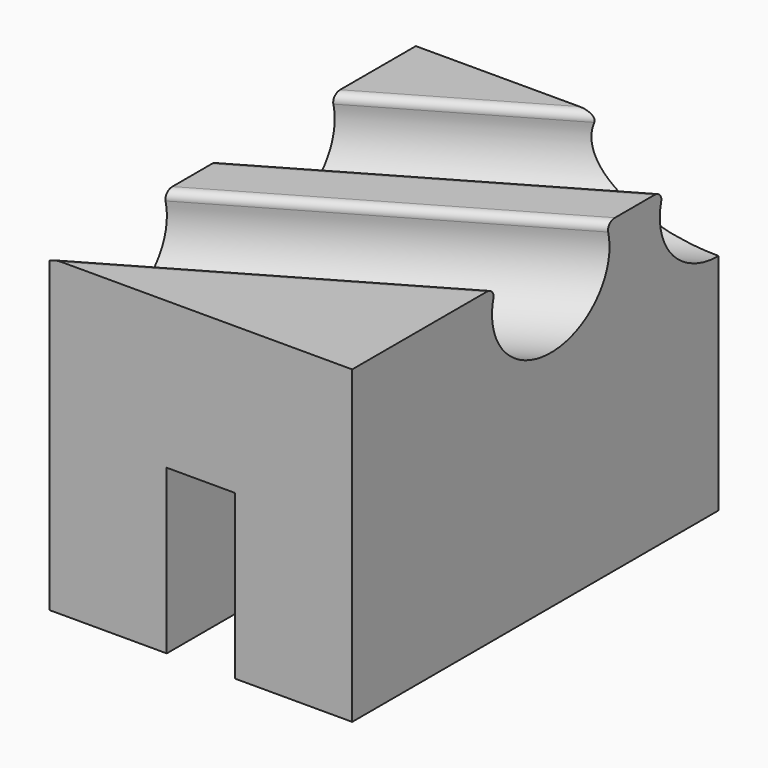
from build123d import *

# Parameters (mm, degrees)
F1_DEPTH      = 24
F1_DEPTH_BACK = 1.5
F4_T1_DEPTH   = 17.3810892057
F4_T3_DEPTH   = 26.4408905281
F4_T5_DEPTH   = 26.4408905281
F4_T7_DEPTH   = 26.4408905281
F6_DEPTH      = 43.7
F7_DEPTH      = 5


# Not quite as in the source:
# - a fillet or chamfer that OpenCascade refuses, or shapes differently, is made with other operations: its cross-section is extruded or revolved along the edge and cut away or added
# - a feature names something its author has since deleted; it is built from what else it names


with BuildPart() as f1:
    # F0 (on Top) → F1 (new body, two sides)
    with BuildSketch(Plane.XY) as f1_sk:
        Polygon((-9.9499136187, 28.9028368274), (-21.5499136187, 28.9028368274), (-21.5499136187, 22.2055737048), align=None)
        Polygon((-1.5499136187, 28.9028368274), (-9.9499136187, 28.9028368274), (-21.5499136187, 22.2055737048), (-21.5499136187, 17.3558314436), align=None)
        Polygon((-1.5499136187, 21.9746335971), (-1.5499136187, 28.9028368274), (-21.5499136187, 17.3558314436), (-21.5499136187, 10.4276282133), align=None)
        Polygon((-1.5499136187, 15.0464303668), (-1.5499136187, 21.9746335971), (-21.5499136187, 10.4276282133), (-21.5499136187, 3.499424983), align=None)
        Polygon((-1.5499136187, -1.3503172782), (-1.5499136187, 10.1966881056), (-21.5499136187, -1.3503172782), align=None)
        Polygon((-1.5499136187, 10.1966881056), (-1.5499136187, 15.0464303668), (-21.5499136187, 3.499424983), (-21.5499136187, -1.3503172782), align=None)
    extrude(amount=-F1_DEPTH)
    extrude(f1_sk.sketch, amount=F1_DEPTH_BACK)

    # F0 (on Top) → F2 (revolve, cut)
    with BuildSketch(Plane.XY):
        Polygon((-21.5499136187, 17.3558314436), (-21.5499136187, 22.2055737048), (-34.8505816362, 14.5264294445), (-32.7505816362, 10.8891227486), align=None)
        Polygon((-1.5499136187, 28.9028368274), (-9.9499136187, 28.9028368274), (-21.5499136187, 22.2055737048), (-21.5499136187, 17.3558314436), align=None)
        Polygon((0, 34.6474221335), (-9.9499136187, 28.9028368274), (-1.5499136187, 28.9028368274), (2.1, 31.0101154376), align=None)
    revolve(axis=Axis((-15.3252908181, 20.9496190931, 0), (-0.8660254038, -0.5, 0)), mode=Mode.SUBTRACT)

    # F0 (on Top) → F3 (revolve, cut)
    with BuildSketch(Plane.XY):
        Polygon((-21.5499136187, -1.3503172782), (-21.5499136187, 3.499424983), (-26.7505816362, 0.4968179032), (-24.6505816362, -3.1404887927), align=None)
        Polygon((-1.5499136187, 10.1966881056), (-1.5499136187, 15.0464303668), (-21.5499136187, 3.499424983), (-21.5499136187, -1.3503172782), align=None)
        Polygon((8.1, 20.6178105922), (-1.5499136187, 15.0464303668), (-1.5499136187, 10.1966881056), (10.2, 16.9805038963), align=None)
    revolve(axis=Axis((-9.3252908181, 10.5573142477, 0), (-0.8660254038, -0.5, 0)), mode=Mode.SUBTRACT)

    # F4: fillet of radius 0.5 on 4 edges, made by hand

    # F4_s2 → F4_t1 (cut)
    with BuildSketch(Plane(origin=(6.9175881272, 3.9938713674, 0), x_dir=(0, 0, 1), z_dir=(-0.8660254038, -0.5, 0))):
        with BuildLine():
            ThreePointArc((1.5, 30.3979327446), (1.3136945255, 30.0085797625), (0.8936170213, 29.9093811487))
            ThreePointArc((0.8936170213, 29.9093811487), (1.2002187189, 29.8304048869), (1.5, 29.7285567925))
            Line((1.5, 29.7285567925), (1.5, 30.3979327446))
        make_face()
    extrude(amount=F4_T1_DEPTH, mode=Mode.SUBTRACT)

    # F4_s4 → F4_t3 (cut)
    with BuildSketch(Plane(origin=(10.8405971764, 6.258821698, 0), x_dir=(0, 0, 1), z_dir=(-0.8660254038, -0.5, 0))):
        with BuildLine():
            ThreePointArc((0.8936170213, 21.7017143379), (1.3136945255, 21.6025157241), (1.5, 21.213162742))
            Line((1.5, 21.213162742), (1.5, 21.8825386941))
            ThreePointArc((1.5, 21.8825386941), (1.2002187189, 21.7806905996), (0.8936170213, 21.7017143379))
        make_face()
    extrude(amount=F4_T3_DEPTH, mode=Mode.SUBTRACT)

    # F4_s6 → F4_t5 (cut)
    with BuildSketch(Plane(origin=(-14.1348766704, -8.1607748506, 0), x_dir=(0, 0, 1), z_dir=(0.8660254038, 0.5, 0))):
        with BuildLine():
            ThreePointArc((1.5, -18.3979327446), (1.3136945255, -18.0085797625), (0.8936170213, -17.9093811487))
            ThreePointArc((0.8936170213, -17.9093811487), (1.2002187189, -17.8304048869), (1.5, -17.7285567925))
            Line((1.5, -17.7285567925), (1.5, -18.3979327446))
        make_face()
    extrude(amount=F4_T5_DEPTH, mode=Mode.SUBTRACT)

    # F4_s8 → F4_t7 (cut)
    with BuildSketch(Plane(origin=(-18.0578857196, -10.4257251812, 0), x_dir=(0, 0, 1), z_dir=(0.8660254038, 0.5, 0))):
        with BuildLine():
            ThreePointArc((0.8936170213, -9.7017143379), (1.3136945255, -9.6025157241), (1.5, -9.213162742))
            Line((1.5, -9.213162742), (1.5, -9.8825386941))
            ThreePointArc((1.5, -9.8825386941), (1.2002187189, -9.7806905996), (0.8936170213, -9.7017143379))
        make_face()
    extrude(amount=F4_T7_DEPTH, mode=Mode.SUBTRACT)

    # F5 (on face) → F6 (cut)
    with BuildSketch(Plane.XZ.offset(1.3503172782)):
        Polygon((-13.7999136187, -26.7), (-9.2999136187, -26.7), (-9.8499136187, -24), (-13.2499136187, -24), align=None)
        Polygon((-9.8499136187, -24), (-9.2999136187, -24), (-9.2999136187, -8.2), (-13.7999136187, -8.2), (-13.7999136187, -24), (-13.2499136187, -24), align=None)
    extrude(amount=-F6_DEPTH, mode=Mode.SUBTRACT)

    # F7 (cut): faces of the model
    f7_faces = [f1.faces().sort_by_distance(p)[0] for p in [
        (-17.6749136187, 13.7762597746, -24),
        (-5.4249136187, 13.7762597746, -24),
    ]]
    extrude(f7_faces, amount=-F7_DEPTH, mode=Mode.SUBTRACT)


solid = f1.part
